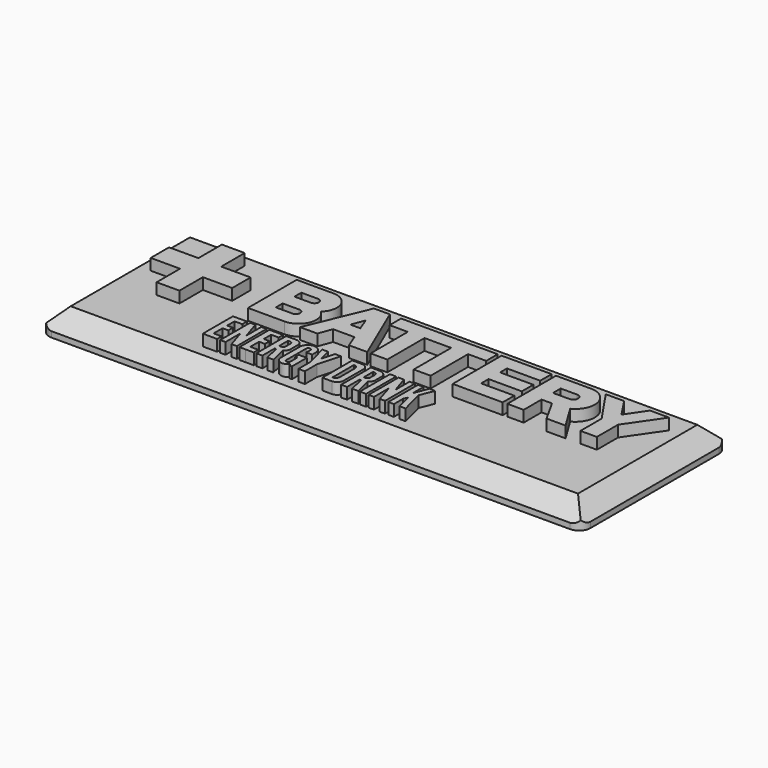
from build123d import *

# Parameters (mm, degrees)
F1_W     = 95.86194
F1_H     = 32.41874
F2_DEPTH = 4
F0_W     = 1.102272
F0_H     = 6.676602
F3_DEPTH = 2
F4_SIZE  = 3
F5_R     = 2


# Not quite as in the source:
# - ends of sketch curves that miss each other by under 0.0002 mm in the source are joined


with BuildPart() as f2:
    # F1 (on Top) → F2 (new body)
    with BuildSketch(Plane.XY):
        Rectangle(F1_W, F1_H)
    extrude(amount=-F2_DEPTH)

    # F0 (on Top) → F3 (join)
    with BuildSketch(Plane.XY):
        Polygon((10.685201, -11.166568), (10.685201, -9.104899), (11.034645, -8.388423), (11.712263, -11.177564), (12.774813, -11.177564), (11.687974, -6.993851), (12.674486, -4.524566), (11.637546, -4.524566), (10.685201, -6.993851), (10.685201, -4.598529), (9.691522, -4.598529), (9.691522, -11.166568), align=None)
        Polygon((-14.218379, -5.553307), (-14.218379, -4.561688), (-15.546487, -4.561688), (-16.649753, -4.561688), (-16.649753, -11.201666), (-15.584869, -11.201666), (-15.546487, -11.201666), (-14.109586, -11.201664), (-14.109586, -10.178552), (-15.546487, -10.178552), (-15.546487, -8.231996), (-14.501253, -8.231996), (-14.501253, -7.193197), (-15.546487, -7.193197), (-15.546487, -5.553307), align=None)
        Polygon((-20.996248, -7.220094), (-22.009499, -7.220094), (-22.009499, -5.580204), (-20.643009, -5.580204), (-20.643009, -4.54335), (-22.009499, -4.54335), (-23.125557, -4.54335), (-23.125557, -11.20937), (-22.009499, -11.20937), (-20.598184, -11.20937), (-20.598184, -10.205448), (-22.009499, -10.205448), (-22.009499, -8.233305), (-20.996248, -8.233305), align=None)
        Polygon((-19.114496, -7.880491), (-18.065056, -11.182474), (-17.12418, -11.182474), (-17.12418, -4.578507), (-18.065056, -4.578507), (-18.065056, -7.880491), (-19.114496, -4.578507), (-20.055372, -4.578507), (-20.055372, -11.191933), (-19.114496, -11.191933), align=None)
        Polygon((38.756302, 3.378407), (42.93097, 9.446433), (39.566087, 9.446433), (37.237538, 6.030508), (34.985757, 9.433639), (31.73602, 9.433639), (35.851477, 3.378407), (35.851477, -1.312167), (38.756302, -1.312167), align=None)
        Polygon((22.123402, 5.404717), (16.231754, 5.404717), (16.231754, 6.942444), (22.121046, 6.942444), (22.121046, 9.466426), (16.231754, 9.466426), (13.260574, 9.466426), (13.260574, -1.365023), (16.231754, -1.365023), (22.113715, -1.365023), (22.113715, 1.207969), (16.231754, 1.207969), (16.231754, 2.865526), (22.123402, 2.865526), align=None)
        with BuildLine():
            Line((25.787262, -1.301718), (25.787262, 2.655426))
            Line((25.787262, 2.655426), (27.643282, 2.655426))
            Line((27.643282, 2.655426), (29.882273, -1.361803))
            Line((29.882273, -1.361803), (33.247153, -1.361803))
            Line((33.247153, -1.361803), (30.598751, 2.975269))
            ThreePointArc((30.598751, 2.975269), (32.4103363087, 6.8284282647), (29.073248, 9.472766))
            Line((29.073248, 9.472766), (25.787262, 9.472766))
            Line((25.787262, 9.472766), (22.894474, 9.472766))
            Line((22.894474, 9.472766), (22.894474, -1.301718))
            Line((22.894474, -1.301718), (25.787262, -1.301718))
        make_face()
        with BuildLine():
            ThreePointArc((28.702216, 6.888434), (29.552999, 6.037651), (28.702216, 5.186868))
            Line((28.702216, 5.186868), (25.787262, 5.186868))
            Line((25.787262, 5.186868), (25.787262, 6.888433))
            Line((25.787262, 6.888433), (28.702216, 6.888434))
        make_face(mode=Mode.SUBTRACT)
        Polygon((-4.543593, 6.920076), (-1.318541, 6.920076), (-1.318541, -1.324541), (1.640139, -1.324541), (1.640139, 6.920076), (6.356691, 6.920076), (6.356691, -1.365023), (9.34993, -1.365023), (9.34993, 6.920076), (12.573806, 6.920076), (12.573806, 9.463974), (-4.543593, 9.463974), align=None)
        Polygon((-6.549783, 9.474202), (-9.364403, 9.474202), (-13.841559, -1.286103), (-10.783831, -1.286103), (-9.897272, 1.093134), (-6.12065, 1.093134), (-5.161718, -1.286103), (-1.941076, -1.286103), align=None)
        Polygon((-8.89409, 3.658743), (-8.00753, 5.956561), (-7.12097, 3.658743), align=None, mode=Mode.SUBTRACT)
        with BuildLine():
            Line((-13.669234, -4.572851), (-13.669234, -11.186124))
            Line((-13.669234, -11.186124), (-12.592697, -11.186124))
            Line((-12.592697, -11.186124), (-12.592697, -8.444917))
            Line((-12.592697, -8.444917), (-12.330348, -8.444917))
            Line((-12.330348, -8.444917), (-11.715184, -11.195171))
            Line((-11.715184, -11.195171), (-10.638648, -11.195171))
            Line((-10.638648, -11.195171), (-11.317137, -8.227792))
            ThreePointArc((-11.317137, -8.227792), (-10.9002695573, -7.8214428415), (-10.747205, -7.259776))
            Line((-10.747205, -7.259776), (-10.747205, -5.568008))
            ThreePointArc((-10.747205, -5.568008), (-11.1191909265, -4.8574968448), (-11.868975, -4.572851))
            Line((-11.868975, -4.572851), (-12.592697, -4.572851))
            Line((-12.592697, -4.572851), (-13.669234, -4.572851))
        make_face()
        with BuildLine():
            Line((-12.592697, -7.485947), (-12.592697, -5.495633))
            Line((-12.592697, -5.495633), (-12.203697, -5.495633))
            ThreePointArc((-12.203697, -5.495633), (-11.9014930079, -5.6375751493), (-11.77851, -5.947978))
            Line((-11.77851, -5.947978), (-11.77851, -6.970276))
            ThreePointArc((-11.77851, -6.970276), (-11.8695181708, -7.3283626359), (-12.203697, -7.485948))
            Line((-12.203697, -7.485948), (-12.592697, -7.485947))
        make_face(mode=Mode.SUBTRACT)
        with BuildLine():
            ThreePointArc((-7.399076, -5.888258), (-8.875504967, -4.4851095908), (-10.2017403449, -6.0309969331))
            Line((-10.2017403449, -6.0309969331), (-10.220403, -10.057698))
            ThreePointArc((-10.220403, -10.057698), (-9.362251328, -11.226319475), (-7.9947400495, -10.7446419666))
            Line((-7.9947400495, -10.7446419666), (-7.794986, -11.174606))
            Line((-7.794986, -11.174606), (-7.372794, -11.174606))
            Line((-7.372794, -11.174606), (-7.372794, -10.138274))
            Line((-7.372794, -10.138274), (-7.372794, -8.718115))
            Line((-7.372794, -8.718115), (-7.372794, -7.874594))
            Line((-7.372794, -7.874594), (-8.782147, -7.874594))
            Line((-8.782147, -7.874594), (-8.782147, -8.719013))
            Line((-8.782147, -8.719013), (-8.436717, -8.719013))
            Line((-8.436717, -8.719013), (-8.436717, -10.139173))
            ThreePointArc((-8.436717, -10.139173), (-8.814452, -10.516908), (-9.192187, -10.139173))
            Line((-9.192187, -10.139173), (-9.171888, -5.759464))
            ThreePointArc((-9.171888, -5.759464), (-8.801896, -5.389472), (-8.431904, -5.759464))
            Line((-8.431904, -5.759464), (-8.431904, -6.646348))
            Line((-8.431904, -6.646348), (-7.399076, -6.646348))
            Line((-7.399076, -6.646348), (-7.399076, -5.888258))
        make_face()
        Polygon((-6.214077, -8.524846), (-6.214077, -11.182225), (-5.073709, -11.182225), (-5.073709, -8.524846), (-3.976373, -4.565674), (-5.019918, -4.565674), (-5.66541, -6.878777), (-6.214077, -4.59795), (-7.257622, -4.59795), align=None)
        with BuildLine():
            Line((-0.942295, -4.564688), (-1.978252, -4.564688))
            Line((-1.978252, -4.564688), (-1.978252, -11.182474))
            Line((-1.978252, -11.182474), (-0.942295, -11.182474))
            Line((-0.942295, -11.182474), (-0.289153, -11.182474))
            ThreePointArc((-0.289153, -11.182474), (0.4752773849, -10.899979208), (0.8723002924, -10.1882700456))
            Line((0.8723002924, -10.1882700456), (0.8723, -5.812317))
            ThreePointArc((0.8723, -5.812317), (0.5738631806, -4.9368440207), (-0.272906, -4.564689))
            Line((-0.272906, -4.564689), (-0.942295, -4.564688))
        make_face()
        with BuildLine():
            Line((-0.942295, -10.224663), (-0.942295, -5.490934))
            ThreePointArc((-0.942295, -5.490934), (-0.4172770722, -5.6844582757), (-0.196351, -6.198547))
            Line((-0.196351, -6.198547), (-0.196351, -9.539989))
            ThreePointArc((-0.196351, -9.539989), (-0.4188610279, -10.0462523896), (-0.942295, -10.224663))
        make_face(mode=Mode.SUBTRACT)
        with BuildLine():
            Line((2.408226, -4.610333), (1.375068, -4.610333))
            Line((1.375068, -4.610333), (1.375068, -11.198422))
            Line((1.375068, -11.198422), (2.408226, -11.198422))
            Line((2.408226, -11.198422), (2.408226, -8.398864))
            Line((2.408226, -8.398864), (2.683109, -8.398864))
            Line((2.683109, -8.398864), (3.275996, -11.183207))
            Line((3.275996, -11.183207), (4.387355, -11.183207))
            Line((4.387355, -11.183207), (3.672757, -8.20107))
            ThreePointArc((3.672757, -8.20107), (4.0811136565, -7.7527620165), (4.228947, -7.164646))
            Line((4.228947, -7.164646), (4.228947, -5.62204))
            ThreePointArc((4.228947, -5.62204), (3.7358562433, -4.892083054), (2.901235, -4.610333))
            Line((2.901235, -4.610333), (2.408226, -4.610333))
        make_face()
        with BuildLine():
            Line((2.408226, -7.492507), (2.408226, -5.448369))
            Line((2.408226, -5.448369), (2.717978, -5.448369))
            ThreePointArc((2.717978, -5.448369), (3.0492312184, -5.6220401722), (3.181911, -5.971735))
            Line((3.181911, -5.971735), (3.181911, -6.981245))
            ThreePointArc((3.181911, -6.981245), (3.0557367204, -7.3195068959), (2.7388579434, -7.492506606))
            Line((2.7388579434, -7.492506606), (2.408226, -7.492507))
        make_face(mode=Mode.SUBTRACT)
        with Locations((5.222403, -7.858779)):
            Rectangle(F0_W, F0_H)
        Polygon((7.185684, -4.574759), (6.228231, -4.574759), (6.228231, -11.19708), (7.185684, -11.19708), (7.185684, -7.88592), (8.18351, -11.178985), (9.122865, -11.178985), (9.122865, -4.574759), (8.18351, -4.574759), (8.18351, -7.668794), align=None)
        Polygon((-33.695532, 11.280453), (-37.741577, 11.280453), (-37.741577, 6.072226), (-42.93097, 6.072226), (-42.93097, 2.011313), (-37.741577, 2.011313), (-37.741577, -3.171464), (-33.695532, -3.171464), (-33.695532, 2.011313), (-28.493563, 2.011313), (-28.493563, 6.072226), (-33.695532, 6.072226), align=None)
        with BuildLine():
            Line((-16.570927, 9.501773), (-23.068154, 9.501773))
            Line((-23.068154, 9.501773), (-23.068154, -1.288558))
            Line((-23.068154, -1.288558), (-16.570927, -1.288558))
            ThreePointArc((-16.570927, -1.288558), (-13.660585936, 0.7192638452), (-14.5042460761, 4.1528729143))
            ThreePointArc((-14.5042460761, 4.1528729143), (-13.7037897685, 7.5358560602), (-16.570927, 9.501773))
        make_face()
        with BuildLine():
            Line((-20.160897, 1.24432), (-20.160897, 2.769849))
            Line((-20.160897, 2.769849), (-17.232369, 2.769849))
            ThreePointArc((-17.232369, 2.769849), (-16.469605, 2.007084), (-17.232369, 1.24432))
            Line((-17.232369, 1.24432), (-20.160897, 1.24432))
        make_face(mode=Mode.SUBTRACT)
        with BuildLine():
            ThreePointArc((-17.232369, 6.896097), (-16.469605, 6.133333), (-17.232369, 5.370569))
            Line((-17.232369, 5.370569), (-20.160897, 5.370569))
            Line((-20.160897, 5.370569), (-20.160897, 6.896097))
            Line((-20.160897, 6.896097), (-17.232369, 6.896097))
        make_face(mode=Mode.SUBTRACT)
    extrude(amount=F3_DEPTH)

    # F4
    f4_edges = [f2.edges().sort_by_distance(p)[0] for p in [
        (0, -16.20937, 0),
        (47.93097, 0, 0),
        (0, 16.20937, 0),
        (-47.93097, 0, 0),
    ]]
    chamfer(f4_edges, length=F4_SIZE)

    # F5
    f5_edges = [f2.edges().sort_by_distance(p)[0] for p in [
        (-47.93097, 16.20937, -3.5),
        (47.93097, 16.20937, -3.5),
        (47.93097, -16.20937, -3.5),
        (-47.93097, -16.20937, -3.5),
    ]]
    fillet(f5_edges, radius=F5_R)


solid = f2.part
